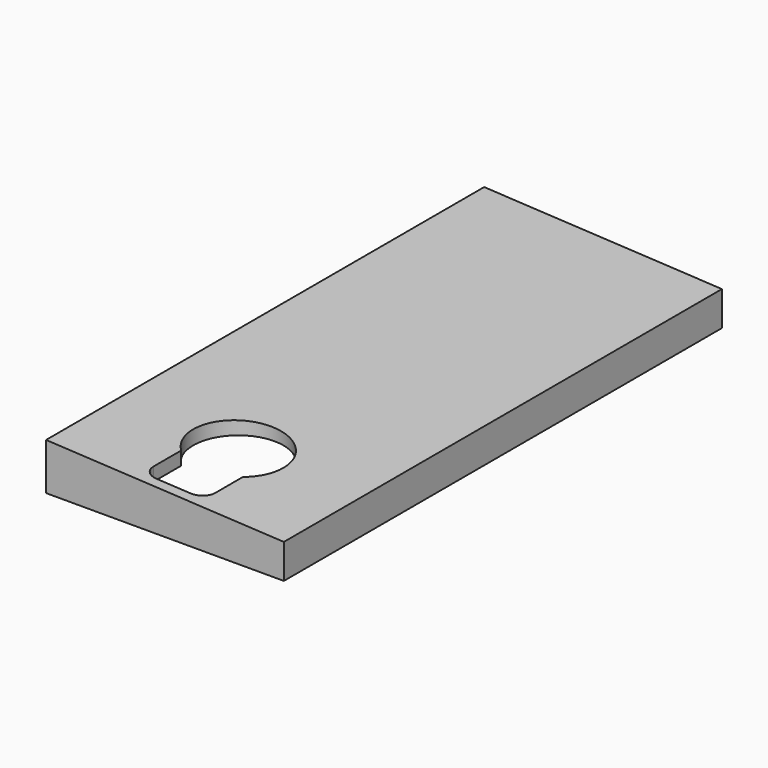
from build123d import *

# Parameters (mm, degrees)
F0_W     = 83.82
F0_H     = 10.16
F1_DEPTH = 193.04
F2_W     = 76.327
F2_H     = 185.547
F3_DEPTH = 10.16
F5_DEPTH = 25.4
F6_R     = 3.81
F7_R     = 4.8259


# Not quite as in the source:
# - a fillet or chamfer is up to 0.001 mm smaller than in the source, because OpenCascade refuses the exact size


with BuildPart() as f1:
    # F0 (on Front) → F1 (new body)
    with BuildSketch(Plane.XZ):
        Polygon((-7.4224442948, 6.35), (-7.4224442948, 0), (76.3975557052, 0), (76.3975557052, 1.9571799405), align=None)
        with Locations((34.4875557052, -5.08)):
            Rectangle(F0_W, F0_H)
    extrude(amount=F1_DEPTH)

    # F2 (on face) → F3 (cut)
    with BuildSketch(Plane(origin=(0, 0, -10.16), x_dir=(1, 0, 0), z_dir=(0, 0, -1))):
        with Locations((34.4875557052, 96.52)):
            Rectangle(F2_W, F2_H)
    extrude(amount=-F3_DEPTH, mode=Mode.SUBTRACT)

    # F4 (on face) → F5 (cut)
    with BuildSketch(Plane(origin=(0, 0, 0), x_dir=(1, 0, 0), z_dir=(0, 0, -1))):
        with BuildLine():
            ThreePointArc((23.6090351158, 172.2802219646), (28.189972413, 146.1460578684), (50.3625557052, 160.7185))
            ThreePointArc((50.3625557052, 160.7185), (49.0599978368, 167.0160832922), (45.3660762946, 172.2802219646))
            ThreePointArc((45.3660762946, 172.2802219646), (34.4875557052, 176.5935), (23.6090351158, 172.2802219646))
        make_face()
        with BuildLine():
            ThreePointArc((23.6090351158, 172.2802219646), (34.4875557052, 176.5935), (45.3660762946, 172.2802219646))
            Line((45.3660762946, 172.2802219646), (45.3660762946, 189.2935))
            Line((45.3660762946, 189.2935), (23.6090351158, 189.2935))
            Line((23.6090351158, 189.2935), (23.6090351158, 172.2802219646))
        make_face()
    extrude(amount=-F5_DEPTH, mode=Mode.SUBTRACT)

    # F6
    f6_edges = [f1.edges().sort_by_distance(p)[0] for p in [
        (59.008566, -189.2935, 0),
        (9.966545, -189.2935, 0),
        (-3.675944, -96.52, 0),
        (72.651056, -96.52, 0),
        (34.487556, -3.7465, 0),
    ]]
    fillet(f6_edges, radius=F6_R)

    # F7 (radius 4.826 in the source; OpenCascade refuses exactly that, so slightly less here)
    f7_edges = [f1.edges().sort_by_distance(p)[0] for p in [
        (45.366076, -189.2935, 1.791735),
        (23.609035, -189.2935, 2.361855),
    ]]
    fillet(f7_edges, radius=F7_R)


solid = f1.part
